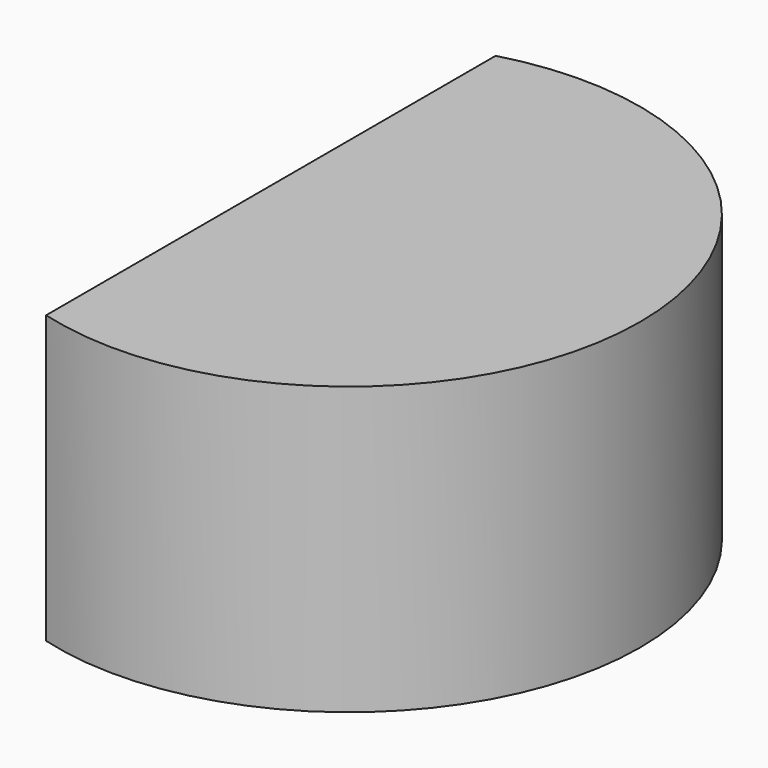
from build123d import *

# Parameters (mm, degrees)
F2_W          = 13.2
F2_H          = 17.7
F3_DEPTH      = 25
F3_DEPTH_BACK = 25
F5_DEPTH      = 0.5
F6_R          = 2
F7_DEPTH      = 5
F8_R          = 1.8
F9_DEPTH      = 4.5
F10_R         = 4.8
F10_R_2       = 1.8
F11_DEPTH     = 1.5
F12_R         = 1.49999
F14_DEPTH     = 1.3
F15_SIZE2     = 0.5
F15_SIZE      = 2


# Not quite as in the source:
# - a fillet or chamfer is up to 0.001 mm smaller than in the source, because OpenCascade refuses the exact size


with BuildPart() as f1:
    # F0 (on Right) → F1 (revolve)
    with BuildSketch(Plane.YZ):
        Polygon((0, 11.7), (0, 17.7), (-18, 17.7), (-18, 0), (-15.1, 0), (-15.1, 1), (-16, 1), (-16, 14.7), (-13.7, 14.7), (-13.7, 16.7), (-5.3, 16.7), (-5.3, 14.7), (-3, 14.7), (-3, 11.7), align=None)
    revolve(axis=Axis((0, 0, 39.4193158346), (0, 0, 1)))

    # F2 (on Front) → F3 (cut, two sides)
    with BuildSketch(Plane.XZ) as f3_sk:
        with Locations((-11.4, 8.85)):
            Rectangle(F2_W, F2_H)
    extrude(amount=F3_DEPTH, mode=Mode.SUBTRACT)
    extrude(f3_sk.sketch, amount=-F3_DEPTH_BACK, mode=Mode.SUBTRACT)

    # F4 (on face) → F5 (join)
    with BuildSketch(Plane(origin=(0, 0, 16.7), x_dir=(1, 0, 0), z_dir=(0, 0, -1))):
        with BuildLine():
            ThreePointArc((-3.8, 13.1624465811), (-4.3031807536, 13.0066381284), (-4.8, 12.8316016148))
            Line((-4.8, 12.8316016148), (-4.8, 2.2472205054))
            ThreePointArc((-4.8, 2.2472205054), (-4.3604724603, 3.012686496), (-3.8, 3.6945906404))
            Line((-3.8, 3.6945906404), (-3.8, 13.1624465811))
        make_face()
        with BuildLine():
            ThreePointArc((-4.8, -12.8316016148), (-4.3031807536, -13.0066381284), (-3.8, -13.1624465811))
            Line((-3.8, -13.1624465811), (-3.8, -3.6945906404))
            ThreePointArc((-3.8, -3.6945906404), (-4.3604724603, -3.012686496), (-4.8, -2.2472205054))
            Line((-4.8, -2.2472205054), (-4.8, -12.8316016148))
        make_face()
    extrude(amount=F5_DEPTH)

    # F6 (on face) → F7 (cut)
    with BuildSketch(Plane(origin=(0, 0, 11.7), x_dir=(1, 0, 0), z_dir=(0, 0, -1))):
        Circle(F6_R)
    extrude(amount=-F7_DEPTH, mode=Mode.SUBTRACT)


with BuildPart() as f9:
    # F8 (on face) → F9 (new body)
    with BuildSketch(Plane(origin=(0, 0, 11.7), x_dir=(1, 0, 0), z_dir=(0, 0, -1))):
        Circle(F8_R)
    extrude(amount=-F9_DEPTH)

    # F10 (on face) → F11 (join)
    with BuildSketch(Plane(origin=(0, 0, 11.7), x_dir=(1, 0, 0), z_dir=(0, 0, -1))):
        Circle(F10_R)
        Circle(F10_R_2, mode=Mode.SUBTRACT)
        Circle(F10_R_2)
    extrude(amount=F11_DEPTH)

    # F12 (radius 1.5 in the source; OpenCascade refuses exactly that, so slightly less here)
    f12_edges = [f9.edges().sort_by_distance(p)[0] for p in [
        (-4.8, 0, 10.2),
    ]]
    fillet(f12_edges, radius=F12_R)


with BuildPart() as f14:
    # F13 (on face) → F14 (new body)
    with BuildSketch(Plane(origin=(0, 0, 16.7), x_dir=(1, 0, 0), z_dir=(0, 0, -1))):
        with BuildLine():
            Line((-3.8, -3.6945906404), (-3.8, -13.1624465811))
            ThreePointArc((-3.8, -13.1624465811), (13.7, 0), (-3.8, 13.1624465811))
            Line((-3.8, 13.1624465811), (-3.8, 3.6945906404))
            ThreePointArc((-3.8, 3.6945906404), (5.3, 0), (-3.8, -3.6945906404))
        make_face()
    extrude(amount=F14_DEPTH)

    # F15
    f15_edges = [f14.edges().sort_by_distance(p)[0] for p in [
        (-3.8, 8.428519, 15.4),
        (-3.8, -8.428519, 15.4),
    ]]
    f15_side = f14.faces().sort_by_distance((-3.474883, -8.428519, 15.4))[0]
    chamfer(f15_edges, length=F15_SIZE, length2=F15_SIZE2, reference=f15_side)


solid = Compound([f1.part, f9.part, f14.part])
